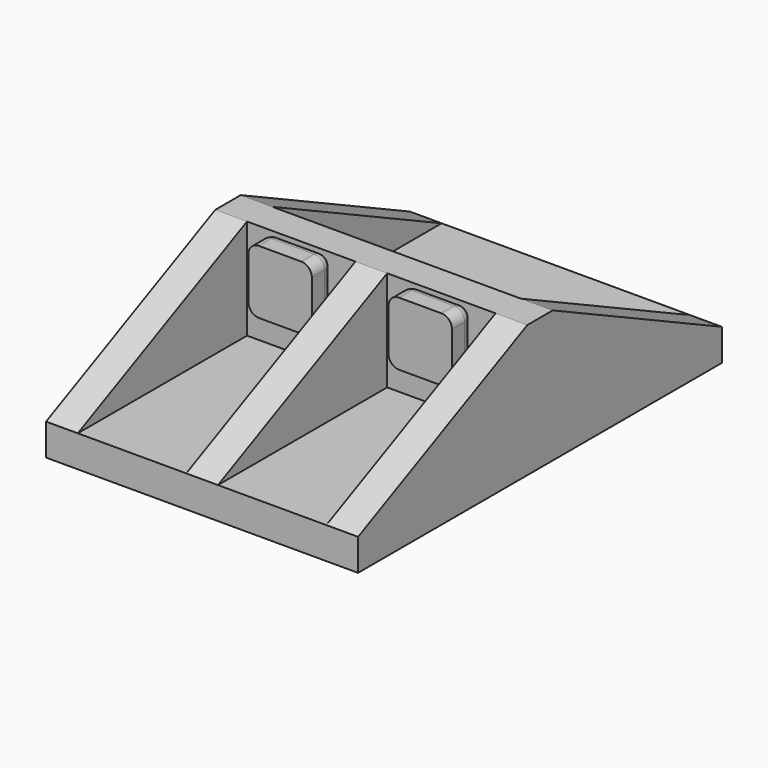
from build123d import *

# Parameters (mm, degrees)
F0_W            = 59
F0_H            = 86
F1_DEPTH        = 6
F3_DEPTH        = 19
F5_DEPTH        = 59.001
F6_W            = 12
F6_H            = 12
F7_DEPTH        = 5
F8_R            = 2
F9_T1_DEPTH     = 8
F9_S5_W         = 2
F9_S5_H         = 2
F9_T6_DEPTH     = 2
F9_S11_W        = 2
F9_S11_H        = 2
F9_T12_DEPTH    = 2
F9_S17_W        = 2
F9_S17_H        = 2
F9_T18_DEPTH    = 2
F9_S23_W        = 2
F9_S23_H        = 2
F9_T24_DEPTH    = 2
F9_S1_T1_DEPTH  = 8
F9_S1_S5_W      = 2
F9_S1_S5_H      = 2
F9_S1_T6_DEPTH  = 2
F9_S1_S11_W     = 2
F9_S1_S11_H     = 2
F9_S1_T12_DEPTH = 2
F9_S1_S17_W     = 2
F9_S1_S17_H     = 2
F9_S1_T18_DEPTH = 2
F9_S1_S23_W     = 2
F9_S1_S23_H     = 2
F9_S1_T24_DEPTH = 2


# Not quite as in the source:
# - a fillet or chamfer that OpenCascade refuses, or shapes differently, is made with other operations: its cross-section is extruded or revolved along the edge and cut away or added


with BuildPart() as f1:
    # F0 (on Top) → F1 (new body)
    with BuildSketch(Plane.XY):
        Rectangle(F0_W, F0_H)
    extrude(amount=F1_DEPTH)

    # F2 (on face) → F3 (join)
    with BuildSketch(Plane.XY.offset(6)):
        Polygon((-23.5, 43), (-29.5, 43), (-29.5, -43), (-23.5, -43), (-23.5, -3), (-3, -3), (-3, -43), (3, -43), (3, -3), (23.5, -3), (23.5, -43), (29.5, -43), (29.5, 43), (23.5, 43), (23.5, 3), (-23.5, 3), align=None)
    extrude(amount=F3_DEPTH)

    # F4 (on face) → F5 (cut, through all)
    with BuildSketch(Plane.YZ.offset(29.5)):
        Polygon((-43, 25), (-43, 6), (-3, 25), align=None)
        Polygon((43, 25), (3, 25), (43, 6), align=None)
    extrude(amount=-F5_DEPTH, mode=Mode.SUBTRACT)


with BuildPart() as f7:
    # F6 (on face) → F7 (new body)
    with BuildSketch(Plane.XZ.offset(3)):
        with Locations((-13.25, 19)):
            Rectangle(F6_W, F6_H)
        with Locations((13.25, 19)):
            Rectangle(F6_W, F6_H)
    extrude(amount=F7_DEPTH)

    # F8
    f8_edges = [f7.edges().sort_by_distance(p)[0] for p in [
        (-7.25, -3, 19),
        (-13.25, -3, 25),
        (-19.25, -3, 19),
        (-13.25, -3, 13),
        (13.25, -3, 13),
        (7.25, -3, 19),
        (19.25, -3, 19),
        (13.25, -3, 25),
    ]]
    fillet(f8_edges, radius=F8_R)

    # F9: fillet of radius 2 on 4 edges, made by hand

    # F9_s2 → F9_t1 (cut)
    with BuildSketch(Plane.XZ.offset(5)):
        with BuildLine():
            ThreePointArc((-7.25, 15), (-7.8357864376, 13.5857864376), (-9.25, 13))
            Line((-9.25, 13), (-7.25, 13))
            Line((-7.25, 13), (-7.25, 15))
        make_face()
        with BuildLine():
            ThreePointArc((-19.25, 15), (-18.6642135624, 13.5857864376), (-17.25, 13))
            Line((-17.25, 13), (-19.25, 13))
            Line((-19.25, 13), (-19.25, 15))
        make_face()
        with BuildLine():
            ThreePointArc((-9.25, 25), (-7.8357864376, 24.4142135624), (-7.25, 23))
            Line((-7.25, 23), (-7.25, 25))
            Line((-7.25, 25), (-9.25, 25))
        make_face()
        with BuildLine():
            ThreePointArc((-17.25, 25), (-18.6642135624, 24.4142135624), (-19.25, 23))
            Line((-19.25, 23), (-19.25, 25))
            Line((-19.25, 25), (-17.25, 25))
        make_face()
    extrude(amount=F9_T1_DEPTH, mode=Mode.SUBTRACT)


with BuildPart() as f9_tool4:
    # F9_s5 → F9_t6 (new body)
    with BuildSketch(Plane.XY.offset(23)):
        with Locations((-18.25, -4)):
            Rectangle(F9_S5_W, F9_S5_H)
    extrude(amount=F9_T6_DEPTH)

    # F9_s7 → F9_t8 (revolve, cut)
    with BuildSketch(Plane(origin=(-17.25, -5, 23), x_dir=(0.7071067812, -0.7071067812, 0), z_dir=(-0.7071067812, -0.7071067812, 0))):
        with BuildLine():
            ThreePointArc((0, -2), (2, 0), (0, 2))
            Line((0, 2), (0, -2))
        make_face()
    revolve(axis=Axis((-17.25, -5, 23), (0, 0, 1)), mode=Mode.SUBTRACT)


with BuildPart() as f7_1:
    add(f7.part)

    # F9_t3: cut F9_tool4
    add(f9_tool4.part, mode=Mode.SUBTRACT)


with BuildPart() as f9_tool10:
    # F9_s11 → F9_t12 (new body)
    with BuildSketch(Plane.XY.offset(23)):
        with Locations((-8.25, -4)):
            Rectangle(F9_S11_W, F9_S11_H)
    extrude(amount=F9_T12_DEPTH)

    # F9_s13 → F9_t14 (revolve, cut)
    with BuildSketch(Plane(origin=(-9.25, -5, 23), x_dir=(-0.7071067812, -0.7071067812, 0), z_dir=(-0.7071067812, 0.7071067812, 0))):
        with BuildLine():
            ThreePointArc((0, -2), (2, 0), (0, 2))
            Line((0, 2), (0, -2))
        make_face()
    revolve(axis=Axis((-9.25, -5, 23), (0, 0, 1)), mode=Mode.SUBTRACT)


with BuildPart() as f7_2:
    add(f7_1.part)

    # F9_t9: cut F9_tool10
    add(f9_tool10.part, mode=Mode.SUBTRACT)


with BuildPart() as f9_tool16:
    # F9_s17 → F9_t18 (new body)
    with BuildSketch(Plane.YZ.offset(-17.25)):
        with Locations((-4, 14)):
            Rectangle(F9_S17_W, F9_S17_H)
    extrude(amount=-F9_T18_DEPTH)

    # F9_s19 → F9_t20 (revolve, cut)
    with BuildSketch(Plane(origin=(-17.25, -5, 15), x_dir=(0, -0.7071067812, 0.7071067812), z_dir=(0, -0.7071067812, -0.7071067812))):
        with BuildLine():
            ThreePointArc((0, -2), (2, 0), (0, 2))
            Line((0, 2), (0, -2))
        make_face()
    revolve(axis=Axis((-17.25, -5, 15), (-1, 0, 0)), mode=Mode.SUBTRACT)


with BuildPart() as f7_3:
    add(f7_2.part)

    # F9_t15: cut F9_tool16
    add(f9_tool16.part, mode=Mode.SUBTRACT)


with BuildPart() as f9_tool22:
    # F9_s23 → F9_t24 (new body)
    with BuildSketch(Plane.YZ.offset(-9.25)):
        with Locations((-4, 14)):
            Rectangle(F9_S23_W, F9_S23_H)
    extrude(amount=F9_T24_DEPTH)

    # F9_s25 → F9_t26 (revolve, cut)
    with BuildSketch(Plane(origin=(-9.25, -5, 15), x_dir=(0, -0.7071067812, 0.7071067812), z_dir=(0, 0.7071067812, 0.7071067812))):
        with BuildLine():
            ThreePointArc((0, -2), (2, 0), (0, 2))
            Line((0, 2), (0, -2))
        make_face()
    revolve(axis=Axis((-9.25, -5, 15), (1, 0, 0)), mode=Mode.SUBTRACT)


with BuildPart() as f7_4:
    add(f7_3.part)

    # F9_t21: cut F9_tool22
    add(f9_tool22.part, mode=Mode.SUBTRACT)

    # F9#s1: fillet of radius 2 on 4 edges, made by hand

    # F9_s1_s2 → F9_s1_t1 (cut)
    with BuildSketch(Plane.XZ.offset(5)):
        with BuildLine():
            ThreePointArc((19.25, 15), (18.6642135624, 13.5857864376), (17.25, 13))
            Line((17.25, 13), (19.25, 13))
            Line((19.25, 13), (19.25, 15))
        make_face()
        with BuildLine():
            ThreePointArc((17.25, 25), (18.6642135624, 24.4142135624), (19.25, 23))
            Line((19.25, 23), (19.25, 25))
            Line((19.25, 25), (17.25, 25))
        make_face()
        with BuildLine():
            ThreePointArc((7.25, 15), (7.8357864376, 13.5857864376), (9.25, 13))
            Line((9.25, 13), (7.25, 13))
            Line((7.25, 13), (7.25, 15))
        make_face()
        with BuildLine():
            ThreePointArc((9.25, 25), (7.8357864376, 24.4142135624), (7.25, 23))
            Line((7.25, 23), (7.25, 25))
            Line((7.25, 25), (9.25, 25))
        make_face()
    extrude(amount=F9_S1_T1_DEPTH, mode=Mode.SUBTRACT)


with BuildPart() as f9_s1_tool4:
    # F9_s1_s5 → F9_s1_t6 (new body)
    with BuildSketch(Plane.XY.offset(23)):
        with Locations((8.25, -4)):
            Rectangle(F9_S1_S5_W, F9_S1_S5_H)
    extrude(amount=F9_S1_T6_DEPTH)

    # F9_s1_s7 → F9_s1_t8 (revolve, cut)
    with BuildSketch(Plane(origin=(9.25, -5, 23), x_dir=(0.7071067812, -0.7071067812, 0), z_dir=(-0.7071067812, -0.7071067812, 0))):
        with BuildLine():
            ThreePointArc((0, -2), (2, 0), (0, 2))
            Line((0, 2), (0, -2))
        make_face()
    revolve(axis=Axis((9.25, -5, 23), (0, 0, 1)), mode=Mode.SUBTRACT)


with BuildPart() as f7_5:
    add(f7_4.part)

    # F9_s1_t3: cut F9_s1_tool4
    add(f9_s1_tool4.part, mode=Mode.SUBTRACT)


with BuildPart() as f9_s1_tool10:
    # F9_s1_s11 → F9_s1_t12 (new body)
    with BuildSketch(Plane.YZ.offset(9.25)):
        with Locations((-4, 14)):
            Rectangle(F9_S1_S11_W, F9_S1_S11_H)
    extrude(amount=-F9_S1_T12_DEPTH)

    # F9_s1_s13 → F9_s1_t14 (revolve, cut)
    with BuildSketch(Plane(origin=(9.25, -5, 15), x_dir=(0, -0.7071067812, 0.7071067812), z_dir=(0, -0.7071067812, -0.7071067812))):
        with BuildLine():
            ThreePointArc((0, -2), (2, 0), (0, 2))
            Line((0, 2), (0, -2))
        make_face()
    revolve(axis=Axis((9.25, -5, 15), (-1, 0, 0)), mode=Mode.SUBTRACT)


with BuildPart() as f7_6:
    add(f7_5.part)

    # F9_s1_t9: cut F9_s1_tool10
    add(f9_s1_tool10.part, mode=Mode.SUBTRACT)


with BuildPart() as f9_s1_tool16:
    # F9_s1_s17 → F9_s1_t18 (new body)
    with BuildSketch(Plane.XY.offset(23)):
        with Locations((18.25, -4)):
            Rectangle(F9_S1_S17_W, F9_S1_S17_H)
    extrude(amount=F9_S1_T18_DEPTH)

    # F9_s1_s19 → F9_s1_t20 (revolve, cut)
    with BuildSketch(Plane(origin=(17.25, -5, 23), x_dir=(-0.7071067812, -0.7071067812, 0), z_dir=(-0.7071067812, 0.7071067812, 0))):
        with BuildLine():
            ThreePointArc((0, -2), (2, 0), (0, 2))
            Line((0, 2), (0, -2))
        make_face()
    revolve(axis=Axis((17.25, -5, 23), (0, 0, 1)), mode=Mode.SUBTRACT)


with BuildPart() as f7_7:
    add(f7_6.part)

    # F9_s1_t15: cut F9_s1_tool16
    add(f9_s1_tool16.part, mode=Mode.SUBTRACT)


with BuildPart() as f9_s1_tool22:
    # F9_s1_s23 → F9_s1_t24 (new body)
    with BuildSketch(Plane.YZ.offset(17.25)):
        with Locations((-4, 14)):
            Rectangle(F9_S1_S23_W, F9_S1_S23_H)
    extrude(amount=F9_S1_T24_DEPTH)

    # F9_s1_s25 → F9_s1_t26 (revolve, cut)
    with BuildSketch(Plane(origin=(17.25, -5, 15), x_dir=(0, -0.7071067812, 0.7071067812), z_dir=(0, 0.7071067812, 0.7071067812))):
        with BuildLine():
            ThreePointArc((0, -2), (2, 0), (0, 2))
            Line((0, 2), (0, -2))
        make_face()
    revolve(axis=Axis((17.25, -5, 15), (1, 0, 0)), mode=Mode.SUBTRACT)


with BuildPart() as f7_8:
    add(f7_7.part)

    # F9_s1_t21: cut F9_s1_tool22
    add(f9_s1_tool22.part, mode=Mode.SUBTRACT)


solid = Compound([f1.part, f7_8.part])
